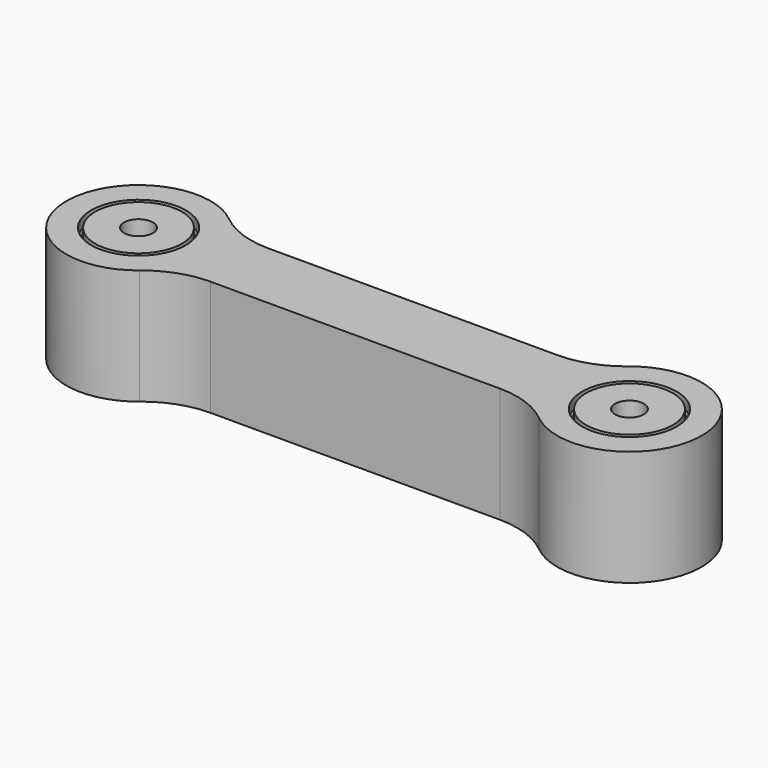
from build123d import *

# Parameters (mm, degrees)
F4_DEPTH = 20


with BuildPart() as f1:
    # F0 (on Front) → F1 (revolve)
    with BuildSketch(Plane.XZ):
        Polygon((-50, 12), (-50, 18), (-52, 16), (-52, 14), align=None)
        Polygon((-46, 10), (-46, 20), (-50, 20), (-50, 18), (-50, 12), (-50, 10), align=None)
        Polygon((-48, 8), (-46, 10), (-50, 10), (-50, 0), (-46.5783654576, 0), (-48, 2.4451902232), align=None)
        Polygon((-45, 11), (-45, 20), (-46, 20), (-46, 10), align=None)
    revolve(axis=Axis((-42.5, 0, 15), (0, 0, -1)))


with BuildPart() as f1b:
    # F0 (on Front) → F1, piece 2 (revolve)
    with BuildSketch(Plane.XZ):
        Polygon((-46, 0), (-46, 9.2928932188), (-47.5, 7.7928932188), (-47.5, 2.5799776423), align=None)
        Polygon((-45, 10.2928932188), (-46, 9.2928932188), (-46, 0), (-45, 0), (-45, 9.2928932188), align=None)
    revolve(axis=Axis((-42.5, 0, 15), (0, 0, -1)))


with BuildPart() as f4:
    # F3 (on Top) → F4 (new body)
    with BuildSketch(Plane.XY):
        with BuildLine():
            ThreePointArc((-31.6746824527, -6.25), (-30.4259271714, -3.2352380638), (-30, 0))
            ThreePointArc((-30, 0), (-30.4259271714, 3.2352380638), (-31.6746824527, 6.25))
            ThreePointArc((-31.6746824527, 6.25), (-32.9666057512, 8.0848249268), (-34.5657727024, 9.6590909091))
            ThreePointArc((-34.5657727024, 9.6590909091), (-55, 0), (-34.5657727024, -9.6590909091))
            ThreePointArc((-34.5657727024, -9.6590909091), (-32.9666057512, -8.0848249268), (-31.6746824527, -6.25))
        make_face()
        with BuildLine():
            ThreePointArc((-31.6746824527, 6.25), (-30.4259271714, 3.2352380638), (-30, 0))
            ThreePointArc((-30, 0), (-30.4259271714, -3.2352380638), (-31.6746824527, -6.25))
            Line((-31.6746824527, -6.25), (-25.0446999453, -6.25))
            Line((-25.0446999453, -6.25), (0, -6.25))
            Line((0, -6.25), (0, 6.25))
            Line((0, 6.25), (-25.0446999453, 6.25))
            Line((-25.0446999453, 6.25), (-31.6746824527, 6.25))
        make_face()
        with BuildLine():
            ThreePointArc((-34.5657727024, 9.6590909091), (-32.9666057512, 8.0848249268), (-31.6746824527, 6.25))
            Line((-31.6746824527, 6.25), (-25.0446999453, 6.25))
            ThreePointArc((-25.0446999453, 6.25), (-30.1011989138, 7.1279669246), (-34.5657727024, 9.6590909091))
        make_face()
        with BuildLine():
            Line((-25.0446999453, -6.25), (-31.6746824527, -6.25))
            ThreePointArc((-31.6746824527, -6.25), (-32.9666057512, -8.0848249268), (-34.5657727024, -9.6590909091))
            ThreePointArc((-34.5657727024, -9.6590909091), (-30.1011989138, -7.1279669246), (-25.0446999453, -6.25))
        make_face()
    extrude(amount=F4_DEPTH)

    # F2 (on Front) → F5 (revolve, cut)
    with BuildSketch(Plane.XZ):
        Polygon((-50, 18), (-50, 20), (-42.5, 20), (-42.5, 20.7), (-50.7, 20.7), (-50.7, 18.2899494937), (-52.7, 16.2899494937), (-52.7, 13.7100505063), (-50.7, 11.7100505063), (-50.7, 0), (-50, 0), (-50, 12), (-52, 14), (-52, 16), align=None)
        Polygon((-42.5, 20), (-50, 20), (-50, 18), (-52, 16), (-52, 14), (-50, 12), (-50, 0), (-42.5, 0), align=None)
    revolve(axis=Axis((-42.5, 0, 10.35), (0, 0, -1)), mode=Mode.SUBTRACT)

    # F6: F4, F1, F1b across face


with BuildPart() as f4_1:
    add(f4.part)
    add(f4.part.mirror(Plane(origin=(0, 0, 10), x_dir=(0, 1, 0), z_dir=(1, 0, 0))))
    add(f1.part.mirror(Plane(origin=(0, 0, 10), x_dir=(0, 1, 0), z_dir=(1, 0, 0))))
    add(f1b.part.mirror(Plane(origin=(0, 0, 10), x_dir=(0, 1, 0), z_dir=(1, 0, 0))))


solid = Compound([f1.part, f1b.part, f4_1.part])
